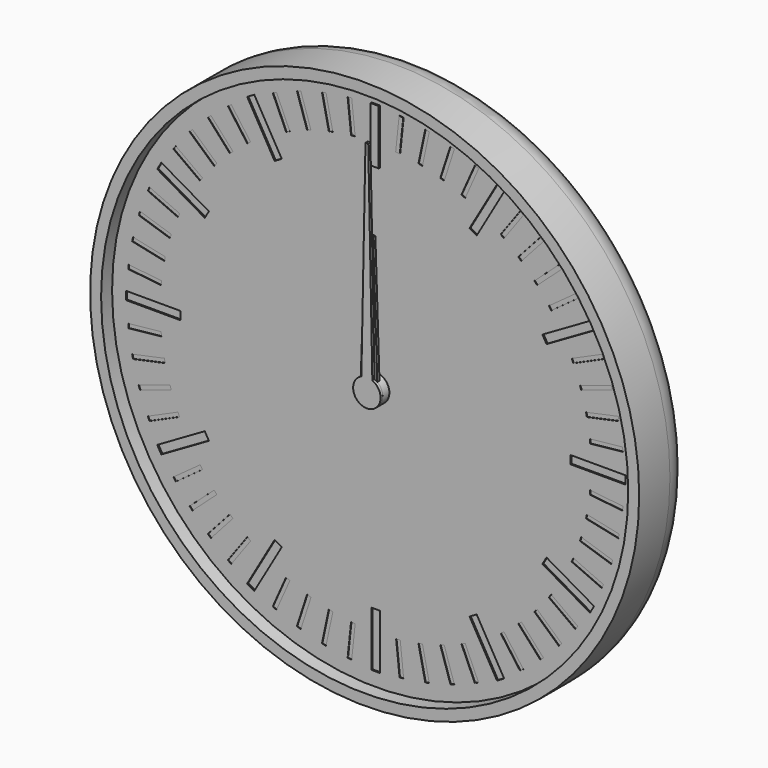
from build123d import *

# Parameters (mm, degrees)
F0_R      = 100
F1_DEPTH  = 24
F2_R      = 10
F3_T      = -4
F4_R      = 5
F4_R_2    = 3
F5_DEPTH  = 2
F6_DEPTH  = 19
F7_DEPTH  = 8
F9_DEPTH  = 4
F11_DEPTH = 4
F12_R     = 5
F12_R_2   = 3
F13_DEPTH = 2
F14_R     = 3
F15_DEPTH = 4
F17_DEPTH = 4
F18_R     = 3
F19_DEPTH = 2
F20_R     = 98
F20_R_2   = 5
F21_DEPTH = 1
F23_R     = 5
F23_R_2   = 3
F24_DEPTH = 2
F25_W     = 3
F25_H     = 20
F25_W_2   = 20
F25_H_2   = 3
F26_DEPTH = 0.5
F27_W     = 1.5
F27_H     = 12
F27_W_2   = 12
F27_H_2   = 1.5
F28_DEPTH = 0.2
F29_DEPTH = 1
F30_DEPTH = 0.4
F31_R     = 5
F31_R_2   = 3
F32_DEPTH = 5
F33_R     = 3
F34_DEPTH = 1
F36_DEPTH = 1


with BuildPart() as f1:
    # F0 (on Front) → F1 (new body)
    with BuildSketch(Plane.XZ):
        Circle(F0_R)
    extrude(amount=F1_DEPTH)

    # F2
    f2_edges = [f1.edges().sort_by_distance(p)[0] for p in [
        (-100, 0, 0),
    ]]
    fillet(f2_edges, radius=F2_R)

    # F3
    f3_openings = [f1.faces().sort_by_distance(p)[0] for p in [
        (0, -24, 0),
    ]]
    offset(amount=F3_T, openings=f3_openings)

    # F4 (on face) → F5 (join)
    with BuildSketch(Plane.XZ.offset(4)):
        Circle(F4_R)
        Circle(F4_R_2, mode=Mode.SUBTRACT)
        with Locations((40, 0)):
            Circle(F4_R)
        with Locations((40, 0)):
            Circle(F4_R_2, mode=Mode.SUBTRACT)
    extrude(amount=F5_DEPTH)


with BuildPart() as f6:
    # F6 (new): a face of the model
    f6_faces = [f1.part.faces().sort_by_distance(p)[0] for p in [
        (0, -4, 0),
    ]]
    extrude(f6_faces, amount=F6_DEPTH)

    # F8 (on face) → F9 (join)
    with BuildSketch(Plane.XZ.offset(6)):
        with BuildLine():
            ThreePointArc((9.2729637667, -1.3794085621), (9.3494561423, -0.6915886375), (9.375, 0))
            ThreePointArc((9.375, 0), (9.3494561423, 0.6915886375), (9.2729637667, 1.3794085621))
            ThreePointArc((9.2729637667, 1.3794085621), (8.9161548403, 2.8970343223), (8.3127812852, 4.3345463782))
            ThreePointArc((8.3127812852, 4.3345463782), (7.5845343223, 5.5104867402), (6.6911892658, 6.566476316))
            ThreePointArc((6.6911892658, 6.566476316), (5.5104867402, 7.5845343223), (4.1773988938, 8.3928519278))
            ThreePointArc((4.1773988938, 8.3928519278), (2.8970343223, 8.9161548403), (1.5536078905, 9.2453733036))
            ThreePointArc((1.5536078905, 9.2453733036), (0, 9.375), (-1.5536078905, 9.2453733036))
            ThreePointArc((-1.5536078905, 9.2453733036), (-2.8970343223, 8.9161548403), (-4.1773988938, 8.3928519278))
            ThreePointArc((-4.1773988938, 8.3928519278), (-5.5104867402, 7.5845343223), (-6.6911892658, 6.566476316))
            ThreePointArc((-6.6911892658, 6.566476316), (-7.5845343223, 5.5104867402), (-8.3127812852, 4.3345463782))
            ThreePointArc((-8.3127812852, 4.3345463782), (-8.9161548403, 2.8970343223), (-9.2729637667, 1.3794085621))
            ThreePointArc((-9.2729637667, 1.3794085621), (-9.375, 0), (-9.2729637667, -1.3794085621))
            ThreePointArc((-9.2729637667, -1.3794085621), (-8.9161548403, -2.8970343223), (-8.3127812852, -4.3345463782))
            ThreePointArc((-8.3127812852, -4.3345463782), (-7.5845343223, -5.5104867402), (-6.6911892658, -6.566476316))
            ThreePointArc((-6.6911892658, -6.566476316), (-5.5104867402, -7.5845343223), (-4.1773988938, -8.3928519278))
            ThreePointArc((-4.1773988938, -8.3928519278), (-2.8970343223, -8.9161548403), (-1.5536078905, -9.2453733036))
            ThreePointArc((-1.5536078905, -9.2453733036), (0, -9.375), (1.5536078905, -9.2453733036))
            ThreePointArc((1.5536078905, -9.2453733036), (2.8970343223, -8.9161548403), (4.1773988938, -8.3928519278))
            ThreePointArc((4.1773988938, -8.3928519278), (5.5104867402, -7.5845343223), (6.6911892658, -6.566476316))
            ThreePointArc((6.6911892658, -6.566476316), (7.5845343223, -5.5104867402), (8.3127812852, -4.3345463782))
            ThreePointArc((8.3127812852, -4.3345463782), (8.9161548403, -2.8970343223), (9.2729637667, -1.3794085621))
        make_face()
        with BuildLine():
            ThreePointArc((8.3127812852, 4.3345463782), (8.9161548403, 2.8970343223), (9.2729637667, 1.3794085621))
            Line((9.2729637667, 1.3794085621), (11.1823199426, 2.3946312492))
            Line((11.1823199426, 2.3946312492), (10.8182678729, 3.515068311))
            Line((10.8182678729, 3.515068311), (10.4542158031, 4.6355053728))
            Line((10.4542158031, 4.6355053728), (8.3127812852, 4.3345463782))
        make_face()
        with BuildLine():
            Line((11.1823199426, -2.3946312492), (9.2729637667, -1.3794085621))
            ThreePointArc((9.2729637667, -1.3794085621), (8.9161548403, -2.8970343223), (8.3127812852, -4.3345463782))
            Line((8.3127812852, -4.3345463782), (10.4542158031, -4.6355053728))
            Line((10.4542158031, -4.6355053728), (10.8182678729, -3.515068311))
            Line((10.8182678729, -3.515068311), (11.1823199426, -2.3946312492))
        make_face()
        with BuildLine():
            ThreePointArc((4.1773988938, 8.3928519278), (5.5104867402, 7.5845343223), (6.6911892658, 6.566476316))
            Line((6.6911892658, 6.566476316), (7.6391579371, 8.5101001246))
            Line((7.6391579371, 8.5101001246), (6.6860572448, 9.202568311))
            Line((6.6860572448, 9.202568311), (5.7329565525, 9.8950364974))
            Line((5.7329565525, 9.8950364974), (4.1773988938, 8.3928519278))
        make_face()
        with BuildLine():
            Line((7.6391579371, -8.5101001246), (6.6911892658, -6.566476316))
            ThreePointArc((6.6911892658, -6.566476316), (5.5104867402, -7.5845343223), (4.1773988938, -8.3928519278))
            Line((4.1773988938, -8.3928519278), (5.7329565525, -9.8950364974))
            Line((5.7329565525, -9.8950364974), (6.6860572448, -9.202568311))
            Line((6.6860572448, -9.202568311), (7.6391579371, -8.5101001246))
        make_face()
        with BuildLine():
            ThreePointArc((-1.5536078905, 9.2453733036), (0, 9.375), (1.5536078905, 9.2453733036))
            Line((1.5536078905, 9.2453733036), (1.1780972451, 11.375))
            Line((1.1780972451, 11.375), (0, 11.375))
            Line((0, 11.375), (-1.1780972451, 11.375))
            Line((-1.1780972451, 11.375), (-1.5536078905, 9.2453733036))
        make_face()
        with BuildLine():
            Line((1.1780972451, -11.375), (1.5536078905, -9.2453733036))
            ThreePointArc((1.5536078905, -9.2453733036), (0, -9.375), (-1.5536078905, -9.2453733036))
            Line((-1.5536078905, -9.2453733036), (-1.1780972451, -11.375))
            Line((-1.1780972451, -11.375), (0, -11.375))
            Line((0, -11.375), (1.1780972451, -11.375))
        make_face()
        with BuildLine():
            ThreePointArc((-6.6911892658, 6.566476316), (-5.5104867402, 7.5845343223), (-4.1773988938, 8.3928519278))
            Line((-4.1773988938, 8.3928519278), (-5.7329565525, 9.8950364974))
            Line((-5.7329565525, 9.8950364974), (-6.6860572448, 9.202568311))
            Line((-6.6860572448, 9.202568311), (-7.6391579371, 8.5101001246))
            Line((-7.6391579371, 8.5101001246), (-6.6911892658, 6.566476316))
        make_face()
        with BuildLine():
            Line((-5.7329565525, -9.8950364974), (-4.1773988938, -8.3928519278))
            ThreePointArc((-4.1773988938, -8.3928519278), (-5.5104867402, -7.5845343223), (-6.6911892658, -6.566476316))
            Line((-6.6911892658, -6.566476316), (-7.6391579371, -8.5101001246))
            Line((-7.6391579371, -8.5101001246), (-6.6860572448, -9.202568311))
            Line((-6.6860572448, -9.202568311), (-5.7329565525, -9.8950364974))
        make_face()
        with BuildLine():
            ThreePointArc((-9.2729637667, 1.3794085621), (-8.9161548403, 2.8970343223), (-8.3127812852, 4.3345463782))
            Line((-8.3127812852, 4.3345463782), (-10.4542158031, 4.6355053728))
            Line((-10.4542158031, 4.6355053728), (-10.8182678729, 3.515068311))
            Line((-10.8182678729, 3.515068311), (-11.1823199426, 2.3946312492))
            Line((-11.1823199426, 2.3946312492), (-9.2729637667, 1.3794085621))
        make_face()
        with BuildLine():
            Line((-10.4542158031, -4.6355053728), (-8.3127812852, -4.3345463782))
            ThreePointArc((-8.3127812852, -4.3345463782), (-8.9161548403, -2.8970343223), (-9.2729637667, -1.3794085621))
            Line((-9.2729637667, -1.3794085621), (-11.1823199426, -2.3946312492))
            Line((-11.1823199426, -2.3946312492), (-10.8182678729, -3.515068311))
            Line((-10.8182678729, -3.515068311), (-10.4542158031, -4.6355053728))
        make_face()
    extrude(amount=F9_DEPTH)

    # F35 (on face) → F36 (join)
    with BuildSketch(Plane.XZ.offset(23)):
        with BuildLine():
            ThreePointArc((-2, 4.582575695), (-2.7386127875, -4.1833001327), (5, 0))
            ThreePointArc((5, 0), (4.1833001327, 2.7386127875), (2, 4.582575695))
            ThreePointArc((2, 4.582575695), (0, 5), (-2, 4.582575695))
        make_face()
        with BuildLine():
            ThreePointArc((-2, 4.582575695), (0, 5), (2, 4.582575695))
            Line((2, 4.582575695), (0.5, 80))
            Line((0.5, 80), (0, 80))
            Line((0, 80), (-0.5, 80))
            Line((-0.5, 80), (-2, 4.582575695))
        make_face()
    extrude(amount=-F36_DEPTH)


with BuildPart() as f7:
    # F7 (new): a face of the model
    f7_faces = [f1.part.faces().sort_by_distance(p)[0] for p in [
        (40, -4, 0),
    ]]
    extrude(f7_faces, amount=F7_DEPTH)

    # F10 (on face) → F11 (join)
    with BuildSketch(Plane.XZ.offset(6)):
        with BuildLine():
            ThreePointArc((68.0831311103, -1.5340704161), (68.1145308291, -0.7673208334), (68.125, 0))
            ThreePointArc((68.125, 0), (68.1145308291, 0.7673208334), (68.0831311103, 1.5340704161))
            ThreePointArc((68.0831311103, 1.5340704161), (67.9709283072, 2.9398630294), (67.7883984907, 4.3382639757))
            ThreePointArc((67.7883984907, 4.3382639757), (67.5104012706, 5.8475163042), (67.1504961426, 7.3393585695))
            ThreePointArc((67.1504961426, 7.3393585695), (66.7484645208, 8.6911029668), (66.2791795135, 10.0209954145))
            ThreePointArc((66.2791795135, 10.0209954145), (65.6934659962, 11.4394680865), (65.0312542109, 12.8238815352))
            ThreePointArc((65.0312542109, 12.8238815352), (64.3569644814, 14.0625), (63.6214342901, 15.2657612676))
            ThreePointArc((63.6214342901, 15.2657612676), (62.7536029668, 16.5314602207), (61.8180263569, 17.747939342))
            ThreePointArc((61.8180263569, 17.747939342), (60.9009482166, 18.8192983038), (59.9313190399, 19.8433401001))
            ThreePointArc((59.9313190399, 19.8433401001), (58.8192983038, 20.9009482166), (57.6512460566, 21.8963270356))
            ThreePointArc((57.6512460566, 21.8963270356), (56.5314602207, 22.7536029668), (55.3701095067, 23.5536697513))
            ThreePointArc((55.3701095067, 23.5536697513), (54.0625, 24.3569644814), (52.7130216036, 25.0877401674))
            ThreePointArc((52.7130216036, 25.0877401674), (51.4394680865, 25.6934659962), (50.137152434, 26.2345910113))
            ThreePointArc((50.137152434, 26.2345910113), (48.6911029668, 26.7484645208), (47.2191771026, 27.1826986696))
            ThreePointArc((47.2191771026, 27.1826986696), (45.8475163042, 27.5104012706), (44.4611531566, 27.7689347566))
            ThreePointArc((44.4611531566, 27.7689347566), (42.9398630294, 27.9709283072), (41.4098199208, 28.0896428028))
            ThreePointArc((41.4098199208, 28.0896428028), (40, 28.125), (38.5901800792, 28.0896428028))
            ThreePointArc((38.5901800792, 28.0896428028), (37.0601369706, 27.9709283072), (35.5388468434, 27.7689347566))
            ThreePointArc((35.5388468434, 27.7689347566), (34.1524836958, 27.5104012706), (32.7808228974, 27.1826986696))
            ThreePointArc((32.7808228974, 27.1826986696), (31.3088970332, 26.7484645208), (29.862847566, 26.2345910113))
            ThreePointArc((29.862847566, 26.2345910113), (28.5605319135, 25.6934659962), (27.2869783964, 25.0877401674))
            ThreePointArc((27.2869783964, 25.0877401674), (25.9375, 24.3569644814), (24.6298904933, 23.5536697513))
            ThreePointArc((24.6298904933, 23.5536697513), (23.4685397793, 22.7536029668), (22.3487539434, 21.8963270356))
            ThreePointArc((22.3487539434, 21.8963270356), (21.1807016962, 20.9009482166), (20.0686809601, 19.8433401001))
            ThreePointArc((20.0686809601, 19.8433401001), (19.0990517834, 18.8192983038), (18.1819736431, 17.747939342))
            ThreePointArc((18.1819736431, 17.747939342), (17.2463970332, 16.5314602207), (16.3785657099, 15.2657612676))
            ThreePointArc((16.3785657099, 15.2657612676), (15.6430355186, 14.0625), (14.9687457891, 12.8238815352))
            ThreePointArc((14.9687457891, 12.8238815352), (14.3065340038, 11.4394680865), (13.7208204865, 10.0209954145))
            ThreePointArc((13.7208204865, 10.0209954145), (13.2515354792, 8.6911029668), (12.8495038574, 7.3393585695))
            ThreePointArc((12.8495038574, 7.3393585695), (12.4895987294, 5.8475163042), (12.2116015093, 4.3382639757))
            ThreePointArc((12.2116015093, 4.3382639757), (12.0290716928, 2.9398630294), (11.9168688897, 1.5340704161))
            ThreePointArc((11.9168688897, 1.5340704161), (11.875, 0), (11.9168688897, -1.5340704161))
            ThreePointArc((11.9168688897, -1.5340704161), (12.0290716928, -2.9398630294), (12.2116015093, -4.3382639757))
            ThreePointArc((12.2116015093, -4.3382639757), (12.4895987294, -5.8475163042), (12.8495038574, -7.3393585695))
            ThreePointArc((12.8495038574, -7.3393585695), (13.2515354792, -8.6911029668), (13.7208204865, -10.0209954145))
            ThreePointArc((13.7208204865, -10.0209954145), (14.3065340038, -11.4394680865), (14.9687457891, -12.8238815352))
            ThreePointArc((14.9687457891, -12.8238815352), (15.6430355186, -14.0625), (16.3785657099, -15.2657612676))
            ThreePointArc((16.3785657099, -15.2657612676), (17.2463970332, -16.5314602207), (18.1819736431, -17.747939342))
            ThreePointArc((18.1819736431, -17.747939342), (19.0990517834, -18.8192983038), (20.0686809601, -19.8433401001))
            ThreePointArc((20.0686809601, -19.8433401001), (21.1807016962, -20.9009482166), (22.3487539434, -21.8963270356))
            ThreePointArc((22.3487539434, -21.8963270356), (23.4685397793, -22.7536029668), (24.6298904933, -23.5536697513))
            ThreePointArc((24.6298904933, -23.5536697513), (25.9375, -24.3569644814), (27.2869783964, -25.0877401674))
            ThreePointArc((27.2869783964, -25.0877401674), (28.5605319135, -25.6934659962), (29.862847566, -26.2345910113))
            ThreePointArc((29.862847566, -26.2345910113), (31.3088970332, -26.7484645208), (32.7808228974, -27.1826986696))
            ThreePointArc((32.7808228974, -27.1826986696), (34.1524836958, -27.5104012706), (35.5388468434, -27.7689347566))
            ThreePointArc((35.5388468434, -27.7689347566), (37.0601369706, -27.9709283072), (38.5901800792, -28.0896428028))
            ThreePointArc((38.5901800792, -28.0896428028), (40, -28.125), (41.4098199208, -28.0896428028))
            ThreePointArc((41.4098199208, -28.0896428028), (42.9398630294, -27.9709283072), (44.4611531566, -27.7689347566))
            ThreePointArc((44.4611531566, -27.7689347566), (45.8475163042, -27.5104012706), (47.2191771026, -27.1826986696))
            ThreePointArc((47.2191771026, -27.1826986696), (48.6911029668, -26.7484645208), (50.137152434, -26.2345910113))
            ThreePointArc((50.137152434, -26.2345910113), (51.4394680865, -25.6934659962), (52.7130216036, -25.0877401674))
            ThreePointArc((52.7130216036, -25.0877401674), (54.0625, -24.3569644814), (55.3701095067, -23.5536697513))
            ThreePointArc((55.3701095067, -23.5536697513), (56.5314602207, -22.7536029668), (57.6512460566, -21.8963270356))
            ThreePointArc((57.6512460566, -21.8963270356), (58.8192983038, -20.9009482166), (59.9313190399, -19.8433401001))
            ThreePointArc((59.9313190399, -19.8433401001), (60.9009482166, -18.8192983038), (61.8180263569, -17.747939342))
            ThreePointArc((61.8180263569, -17.747939342), (62.7536029668, -16.5314602207), (63.6214342901, -15.2657612676))
            ThreePointArc((63.6214342901, -15.2657612676), (64.3569644814, -14.0625), (65.0312542109, -12.8238815352))
            ThreePointArc((65.0312542109, -12.8238815352), (65.6934659962, -11.4394680865), (66.2791795135, -10.0209954145))
            ThreePointArc((66.2791795135, -10.0209954145), (66.7484645208, -8.6911029668), (67.1504961426, -7.3393585695))
            ThreePointArc((67.1504961426, -7.3393585695), (67.5104012706, -5.8475163042), (67.7883984907, -4.3382639757))
            ThreePointArc((67.7883984907, -4.3382639757), (67.9709283072, -2.9398630294), (68.0831311103, -1.5340704161))
        make_face()
        with BuildLine():
            ThreePointArc((68.0831311103, 1.5340704161), (68.1145308291, 0.7673208334), (68.125, 0))
            ThreePointArc((68.125, 0), (68.1145308291, -0.7673208334), (68.0831311103, -1.5340704161))
            Line((68.0831311103, -1.5340704161), (70.1019552834, -1.1780972451))
            Line((70.1019552834, -1.1780972451), (70.1019552834, 0))
            Line((70.1019552834, 0), (70.1019552834, 1.1780972451))
            Line((70.1019552834, 1.1780972451), (68.0831311103, 1.5340704161))
        make_face()
        with BuildLine():
            ThreePointArc((67.1504961426, 7.3393585695), (67.5104012706, 5.8475163042), (67.7883984907, 4.3382639757))
            Line((67.7883984907, 4.3382639757), (69.689095528, 5.1061954262))
            Line((69.689095528, 5.1061954262), (69.4441553378, 6.2585484199))
            Line((69.4441553378, 6.2585484199), (69.1992151476, 7.4109014136))
            Line((69.1992151476, 7.4109014136), (67.1504961426, 7.3393585695))
        make_face()
        with BuildLine():
            Line((69.689095528, -5.1061954262), (67.7883984907, -4.3382639757))
            ThreePointArc((67.7883984907, -4.3382639757), (67.5104012706, -5.8475163042), (67.1504961426, -7.3393585695))
            Line((67.1504961426, -7.3393585695), (69.1992151476, -7.4109014136))
            Line((69.1992151476, -7.4109014136), (69.4441553378, -6.2585484199))
            Line((69.4441553378, -6.2585484199), (69.689095528, -5.1061954262))
        make_face()
        with BuildLine():
            ThreePointArc((65.0312542109, 12.8238815352), (65.6934659962, 11.4394680865), (66.2791795135, 10.0209954145))
            Line((66.2791795135, 10.0209954145), (67.978679834, 11.1673228551))
            Line((67.978679834, 11.1673228551), (67.4995045153, 12.243568242))
            Line((67.4995045153, 12.243568242), (67.0203291966, 13.3198136289))
            Line((67.0203291966, 13.3198136289), (65.0312542109, 12.8238815352))
        make_face()
        with BuildLine():
            Line((67.978679834, -11.1673228551), (66.2791795135, -10.0209954145))
            ThreePointArc((66.2791795135, -10.0209954145), (65.6934659962, -11.4394680865), (65.0312542109, -12.8238815352))
            Line((65.0312542109, -12.8238815352), (67.0203291966, -13.3198136289))
            Line((67.0203291966, -13.3198136289), (67.4995045153, -12.243568242))
            Line((67.4995045153, -12.243568242), (67.978679834, -11.1673228551))
        make_face()
        with BuildLine():
            ThreePointArc((61.8180263569, 17.747939342), (62.7536029668, 16.5314602207), (63.6214342901, 15.2657612676))
            Line((63.6214342901, 15.2657612676), (65.0454615746, 16.7403846884))
            Line((65.0454615746, 16.7403846884), (64.3529933881, 17.6934853807))
            Line((64.3529933881, 17.6934853807), (63.6605252017, 18.646586073))
            Line((63.6605252017, 18.646586073), (61.8180263569, 17.747939342))
        make_face()
        with BuildLine():
            Line((65.0454615746, -16.7403846884), (63.6214342901, -15.2657612676))
            ThreePointArc((63.6214342901, -15.2657612676), (62.7536029668, -16.5314602207), (61.8180263569, -17.747939342))
            Line((61.8180263569, -17.747939342), (63.6605252017, -18.646586073))
            Line((63.6605252017, -18.646586073), (64.3529933881, -17.6934853807))
            Line((64.3529933881, -17.6934853807), (65.0454615746, -16.7403846884))
        make_face()
        with BuildLine():
            ThreePointArc((57.6512460566, 21.8963270356), (58.8192983038, 20.9009482166), (59.9313190399, 19.8433401001))
            Line((59.9313190399, 19.8433401001), (61.0176364629, 21.5818113816))
            Line((61.0176364629, 21.5818113816), (60.1421395913, 22.3701123056))
            Line((60.1421395913, 22.3701123056), (59.2666427197, 23.1584132295))
            Line((59.2666427197, 23.1584132295), (57.6512460566, 21.8963270356))
        make_face()
        with BuildLine():
            Line((61.0176364629, -21.5818113816), (59.9313190399, -19.8433401001))
            ThreePointArc((59.9313190399, -19.8433401001), (58.8192983038, -20.9009482166), (57.6512460566, -21.8963270356))
            Line((57.6512460566, -21.8963270356), (59.2666427197, -23.1584132295))
            Line((59.2666427197, -23.1584132295), (60.1421395913, -22.3701123056))
            Line((60.1421395913, -22.3701123056), (61.0176364629, -21.5818113816))
        make_face()
        with BuildLine():
            ThreePointArc((52.7130216036, 25.0877401674), (54.0625, 24.3569644814), (55.3701095067, 23.5536697513))
            Line((55.3701095067, 23.5536697513), (56.0712397841, 25.4800093564))
            Line((56.0712397841, 25.4800093564), (55.0509776417, 26.069057979))
            Line((55.0509776417, 26.069057979), (54.0307154993, 26.6581066015))
            Line((54.0307154993, 26.6581066015), (52.7130216036, 25.0877401674))
        make_face()
        with BuildLine():
            Line((56.0712397841, -25.4800093564), (55.3701095067, -23.5536697513))
            ThreePointArc((55.3701095067, -23.5536697513), (54.0625, -24.3569644814), (52.7130216036, -25.0877401674))
            Line((52.7130216036, -25.0877401674), (54.0307154993, -26.6581066015))
            Line((54.0307154993, -26.6581066015), (55.0509776417, -26.069057979))
            Line((55.0509776417, -26.069057979), (56.0712397841, -25.4800093564))
        make_face()
        with BuildLine():
            ThreePointArc((47.2191771026, 27.1826986696), (48.6911029668, 26.7484645208), (50.137152434, 26.2345910113))
            Line((50.137152434, 26.2345910113), (50.4224528082, 28.2646086557))
            Line((50.4224528082, 28.2646086557), (49.3020157465, 28.6286607255))
            Line((49.3020157465, 28.6286607255), (48.1815786847, 28.9927127952))
            Line((48.1815786847, 28.9927127952), (47.2191771026, 27.1826986696))
        make_face()
        with BuildLine():
            Line((50.4224528082, -28.2646086557), (50.137152434, -26.2345910113))
            ThreePointArc((50.137152434, -26.2345910113), (48.6911029668, -26.7484645208), (47.2191771026, -27.1826986696))
            Line((47.2191771026, -27.1826986696), (48.1815786847, -28.9927127952))
            Line((48.1815786847, -28.9927127952), (49.3020157465, -28.6286607255))
            Line((49.3020157465, -28.6286607255), (50.4224528082, -28.2646086557))
        make_face()
        with BuildLine():
            ThreePointArc((41.4098199208, 28.0896428028), (42.9398630294, 27.9709283072), (44.4611531566, 27.7689347566))
            Line((44.4611531566, 27.7689347566), (44.3181546322, 29.8139089281))
            Line((44.3181546322, 29.8139089281), (43.1465111271, 29.9370536227))
            Line((43.1465111271, 29.9370536227), (41.974867622, 30.0601983173))
            Line((41.974867622, 30.0601983173), (41.4098199208, 28.0896428028))
        make_face()
        with BuildLine():
            Line((44.3181546322, -29.8139089281), (44.4611531566, -27.7689347566))
            ThreePointArc((44.4611531566, -27.7689347566), (42.9398630294, -27.9709283072), (41.4098199208, -28.0896428028))
            Line((41.4098199208, -28.0896428028), (41.974867622, -30.0601983173))
            Line((41.974867622, -30.0601983173), (43.1465111271, -29.9370536227))
            Line((43.1465111271, -29.9370536227), (44.3181546322, -29.8139089281))
        make_face()
        with BuildLine():
            ThreePointArc((35.5388468434, 27.7689347566), (37.0601369706, 27.9709283072), (38.5901800792, 28.0896428028))
            Line((38.5901800792, 28.0896428028), (38.025132378, 30.0601983173))
            Line((38.025132378, 30.0601983173), (36.8534888729, 29.9370536227))
            Line((36.8534888729, 29.9370536227), (35.6818453678, 29.8139089281))
            Line((35.6818453678, 29.8139089281), (35.5388468434, 27.7689347566))
        make_face()
        with BuildLine():
            Line((38.025132378, -30.0601983173), (38.5901800792, -28.0896428028))
            ThreePointArc((38.5901800792, -28.0896428028), (37.0601369706, -27.9709283072), (35.5388468434, -27.7689347566))
            Line((35.5388468434, -27.7689347566), (35.6818453678, -29.8139089281))
            Line((35.6818453678, -29.8139089281), (36.8534888729, -29.9370536227))
            Line((36.8534888729, -29.9370536227), (38.025132378, -30.0601983173))
        make_face()
        with BuildLine():
            ThreePointArc((29.862847566, 26.2345910113), (31.3088970332, 26.7484645208), (32.7808228974, 27.1826986696))
            Line((32.7808228974, 27.1826986696), (31.8184213153, 28.9927127952))
            Line((31.8184213153, 28.9927127952), (30.6979842535, 28.6286607255))
            Line((30.6979842535, 28.6286607255), (29.5775471918, 28.2646086557))
            Line((29.5775471918, 28.2646086557), (29.862847566, 26.2345910113))
        make_face()
        with BuildLine():
            Line((31.8184213153, -28.9927127952), (32.7808228974, -27.1826986696))
            ThreePointArc((32.7808228974, -27.1826986696), (31.3088970332, -26.7484645208), (29.862847566, -26.2345910113))
            Line((29.862847566, -26.2345910113), (29.5775471918, -28.2646086557))
            Line((29.5775471918, -28.2646086557), (30.6979842535, -28.6286607255))
            Line((30.6979842535, -28.6286607255), (31.8184213153, -28.9927127952))
        make_face()
        with BuildLine():
            ThreePointArc((24.6298904933, 23.5536697513), (25.9375, 24.3569644814), (27.2869783964, 25.0877401674))
            Line((27.2869783964, 25.0877401674), (25.9692845007, 26.6581066015))
            Line((25.9692845007, 26.6581066015), (24.9490223583, 26.069057979))
            Line((24.9490223583, 26.069057979), (23.9287602159, 25.4800093564))
            Line((23.9287602159, 25.4800093564), (24.6298904933, 23.5536697513))
        make_face()
        with BuildLine():
            Line((25.9692845007, -26.6581066015), (27.2869783964, -25.0877401674))
            ThreePointArc((27.2869783964, -25.0877401674), (25.9375, -24.3569644814), (24.6298904933, -23.5536697513))
            Line((24.6298904933, -23.5536697513), (23.9287602159, -25.4800093564))
            Line((23.9287602159, -25.4800093564), (24.9490223583, -26.069057979))
            Line((24.9490223583, -26.069057979), (25.9692845007, -26.6581066015))
        make_face()
        with BuildLine():
            ThreePointArc((20.0686809601, 19.8433401001), (21.1807016962, 20.9009482166), (22.3487539434, 21.8963270356))
            Line((22.3487539434, 21.8963270356), (20.7333572803, 23.1584132295))
            Line((20.7333572803, 23.1584132295), (19.8578604087, 22.3701123056))
            Line((19.8578604087, 22.3701123056), (18.9823635371, 21.5818113816))
            Line((18.9823635371, 21.5818113816), (20.0686809601, 19.8433401001))
        make_face()
        with BuildLine():
            Line((20.7333572803, -23.1584132295), (22.3487539434, -21.8963270356))
            ThreePointArc((22.3487539434, -21.8963270356), (21.1807016962, -20.9009482166), (20.0686809601, -19.8433401001))
            Line((20.0686809601, -19.8433401001), (18.9823635371, -21.5818113816))
            Line((18.9823635371, -21.5818113816), (19.8578604087, -22.3701123056))
            Line((19.8578604087, -22.3701123056), (20.7333572803, -23.1584132295))
        make_face()
        with BuildLine():
            ThreePointArc((16.3785657099, 15.2657612676), (17.2463970332, 16.5314602207), (18.1819736431, 17.747939342))
            Line((18.1819736431, 17.747939342), (16.3394747983, 18.646586073))
            Line((16.3394747983, 18.646586073), (15.6470066119, 17.6934853807))
            Line((15.6470066119, 17.6934853807), (14.9545384254, 16.7403846884))
            Line((14.9545384254, 16.7403846884), (16.3785657099, 15.2657612676))
        make_face()
        with BuildLine():
            Line((16.3394747983, -18.646586073), (18.1819736431, -17.747939342))
            ThreePointArc((18.1819736431, -17.747939342), (17.2463970332, -16.5314602207), (16.3785657099, -15.2657612676))
            Line((16.3785657099, -15.2657612676), (14.9545384254, -16.7403846884))
            Line((14.9545384254, -16.7403846884), (15.6470066119, -17.6934853807))
            Line((15.6470066119, -17.6934853807), (16.3394747983, -18.646586073))
        make_face()
        with BuildLine():
            ThreePointArc((13.7208204865, 10.0209954145), (14.3065340038, 11.4394680865), (14.9687457891, 12.8238815352))
            Line((14.9687457891, 12.8238815352), (12.9796708034, 13.3198136289))
            Line((12.9796708034, 13.3198136289), (12.5004954847, 12.243568242))
            Line((12.5004954847, 12.243568242), (12.021320166, 11.1673228551))
            Line((12.021320166, 11.1673228551), (13.7208204865, 10.0209954145))
        make_face()
        with BuildLine():
            Line((12.9796708034, -13.3198136289), (14.9687457891, -12.8238815352))
            ThreePointArc((14.9687457891, -12.8238815352), (14.3065340038, -11.4394680865), (13.7208204865, -10.0209954145))
            Line((13.7208204865, -10.0209954145), (12.021320166, -11.1673228551))
            Line((12.021320166, -11.1673228551), (12.5004954847, -12.243568242))
            Line((12.5004954847, -12.243568242), (12.9796708034, -13.3198136289))
        make_face()
        with BuildLine():
            ThreePointArc((12.2116015093, 4.3382639757), (12.4895987294, 5.8475163042), (12.8495038574, 7.3393585695))
            Line((12.8495038574, 7.3393585695), (10.8007848524, 7.4109014136))
            Line((10.8007848524, 7.4109014136), (10.5558446622, 6.2585484199))
            Line((10.5558446622, 6.2585484199), (10.310904472, 5.1061954262))
            Line((10.310904472, 5.1061954262), (12.2116015093, 4.3382639757))
        make_face()
        with BuildLine():
            Line((10.8007848524, -7.4109014136), (12.8495038574, -7.3393585695))
            ThreePointArc((12.8495038574, -7.3393585695), (12.4895987294, -5.8475163042), (12.2116015093, -4.3382639757))
            Line((12.2116015093, -4.3382639757), (10.310904472, -5.1061954262))
            Line((10.310904472, -5.1061954262), (10.5558446622, -6.2585484199))
            Line((10.5558446622, -6.2585484199), (10.8007848524, -7.4109014136))
        make_face()
        with BuildLine():
            ThreePointArc((11.9168688897, -1.5340704161), (11.875, 0), (11.9168688897, 1.5340704161))
            Line((11.9168688897, 1.5340704161), (9.8980447166, 1.1780972451))
            Line((9.8980447166, 1.1780972451), (9.8980447166, 0))
            Line((9.8980447166, 0), (9.8980447166, -1.1780972451))
            Line((9.8980447166, -1.1780972451), (11.9168688897, -1.5340704161))
        make_face()
    extrude(amount=F11_DEPTH)

    # F16 (on face) → F17 (join)
    with BuildSketch(Plane.XZ.offset(12)):
        with BuildLine():
            ThreePointArc((47.4288750323, -1.0304444454), (47.4821976298, -0.5164480894), (47.5, 0))
            ThreePointArc((47.5, 0), (47.4821976298, 0.5164480894), (47.4288750323, 1.0304444454))
            ThreePointArc((47.4288750323, 1.0304444454), (47.1329238722, 2.3176274578), (46.6157661985, 3.532936117))
            ThreePointArc((46.6157661985, 3.532936117), (46.0676274578, 4.4083893922), (45.4044061018, 5.2002302532))
            ThreePointArc((45.4044061018, 5.2002302532), (44.4083893922, 6.0676274578), (43.2756595386, 6.7468551628))
            ThreePointArc((43.2756595386, 6.7468551628), (42.3176274578, 7.1329238722), (41.3156377295, 7.3837048536))
            ThreePointArc((41.3156377295, 7.3837048536), (40, 7.5), (38.6843622705, 7.3837048536))
            ThreePointArc((38.6843622705, 7.3837048536), (37.6823725422, 7.1329238722), (36.7243404614, 6.7468551628))
            ThreePointArc((36.7243404614, 6.7468551628), (35.5916106078, 6.0676274578), (34.5955938982, 5.2002302532))
            ThreePointArc((34.5955938982, 5.2002302532), (33.9323725422, 4.4083893922), (33.3842338015, 3.532936117))
            ThreePointArc((33.3842338015, 3.532936117), (32.8670761278, 2.3176274578), (32.5711249677, 1.0304444454))
            ThreePointArc((32.5711249677, 1.0304444454), (32.5, 0), (32.5711249677, -1.0304444454))
            ThreePointArc((32.5711249677, -1.0304444454), (32.8670761278, -2.3176274578), (33.3842338015, -3.532936117))
            ThreePointArc((33.3842338015, -3.532936117), (33.9323725422, -4.4083893922), (34.5955938982, -5.2002302532))
            ThreePointArc((34.5955938982, -5.2002302532), (35.5916106078, -6.0676274578), (36.7243404614, -6.7468551628))
            ThreePointArc((36.7243404614, -6.7468551628), (37.6823725422, -7.1329238722), (38.6843622705, -7.3837048536))
            ThreePointArc((38.6843622705, -7.3837048536), (40, -7.5), (41.3156377295, -7.3837048536))
            ThreePointArc((41.3156377295, -7.3837048536), (42.3176274578, -7.1329238722), (43.2756595386, -6.7468551628))
            ThreePointArc((43.2756595386, -6.7468551628), (44.4083893922, -6.0676274578), (45.4044061018, -5.2002302532))
            ThreePointArc((45.4044061018, -5.2002302532), (46.0676274578, -4.4083893922), (46.6157661985, -3.532936117))
            ThreePointArc((46.6157661985, -3.532936117), (47.1329238722, -2.3176274578), (47.4288750323, -1.0304444454))
        make_face()
        with BuildLine():
            ThreePointArc((46.6157661985, 3.532936117), (47.1329238722, 2.3176274578), (47.4288750323, 1.0304444454))
            Line((47.4288750323, 1.0304444454), (49.3262785606, 2.0393117971))
            Line((49.3262785606, 2.0393117971), (48.743795249, 3.832011096))
            Line((48.743795249, 3.832011096), (46.6157661985, 3.532936117))
        make_face()
        with BuildLine():
            Line((49.3262785606, -2.0393117971), (47.4288750323, -1.0304444454))
            ThreePointArc((47.4288750323, -1.0304444454), (47.1329238722, -2.3176274578), (46.6157661985, -3.532936117))
            Line((46.6157661985, -3.532936117), (48.743795249, -3.832011096))
            Line((48.743795249, -3.832011096), (49.3262785606, -2.0393117971))
        make_face()
        with BuildLine():
            ThreePointArc((43.2756595386, 6.7468551628), (44.4083893922, 6.0676274578), (45.4044061018, 5.2002302532))
            Line((45.4044061018, 5.2002302532), (46.3464404506, 7.1316868974))
            Line((46.3464404506, 7.1316868974), (44.8214793429, 8.2396359957))
            Line((44.8214793429, 8.2396359957), (43.2756595386, 6.7468551628))
        make_face()
        with BuildLine():
            Line((46.3464404506, -7.1316868974), (45.4044061018, -5.2002302532))
            ThreePointArc((45.4044061018, -5.2002302532), (44.4083893922, -6.0676274578), (43.2756595386, -6.7468551628))
            Line((43.2756595386, -6.7468551628), (44.8214793429, -8.2396359957))
            Line((44.8214793429, -8.2396359957), (46.3464404506, -7.1316868974))
        make_face()
        with BuildLine():
            ThreePointArc((38.6843622705, 7.3837048536), (40, 7.5), (41.3156377295, 7.3837048536))
            Line((41.3156377295, 7.3837048536), (40.9424777961, 9.5))
            Line((40.9424777961, 9.5), (39.0575222039, 9.5))
            Line((39.0575222039, 9.5), (38.6843622705, 7.3837048536))
        make_face()
        with BuildLine():
            Line((40.9424777961, -9.5), (41.3156377295, -7.3837048536))
            ThreePointArc((41.3156377295, -7.3837048536), (40, -7.5), (38.6843622705, -7.3837048536))
            Line((38.6843622705, -7.3837048536), (39.0575222039, -9.5))
            Line((39.0575222039, -9.5), (40.9424777961, -9.5))
        make_face()
        with BuildLine():
            ThreePointArc((34.5955938982, 5.2002302532), (35.5916106078, 6.0676274578), (36.7243404614, 6.7468551628))
            Line((36.7243404614, 6.7468551628), (35.1785206571, 8.2396359957))
            Line((35.1785206571, 8.2396359957), (33.6535595494, 7.1316868974))
            Line((33.6535595494, 7.1316868974), (34.5955938982, 5.2002302532))
        make_face()
        with BuildLine():
            Line((35.1785206571, -8.2396359957), (36.7243404614, -6.7468551628))
            ThreePointArc((36.7243404614, -6.7468551628), (35.5916106078, -6.0676274578), (34.5955938982, -5.2002302532))
            Line((34.5955938982, -5.2002302532), (33.6535595494, -7.1316868974))
            Line((33.6535595494, -7.1316868974), (35.1785206571, -8.2396359957))
        make_face()
        with BuildLine():
            ThreePointArc((32.5711249677, 1.0304444454), (32.8670761278, 2.3176274578), (33.3842338015, 3.532936117))
            Line((33.3842338015, 3.532936117), (31.256204751, 3.832011096))
            Line((31.256204751, 3.832011096), (30.6737214394, 2.0393117971))
            Line((30.6737214394, 2.0393117971), (32.5711249677, 1.0304444454))
        make_face()
        with BuildLine():
            Line((31.256204751, -3.832011096), (33.3842338015, -3.532936117))
            ThreePointArc((33.3842338015, -3.532936117), (32.8670761278, -2.3176274578), (32.5711249677, -1.0304444454))
            Line((32.5711249677, -1.0304444454), (30.6737214394, -2.0393117971))
            Line((30.6737214394, -2.0393117971), (31.256204751, -3.832011096))
        make_face()
    extrude(amount=F17_DEPTH)

    # F18 (on face) → F19 (join)
    with BuildSketch(Plane.XZ.offset(16)):
        with Locations((40, 0)):
            Circle(F18_R)
    extrude(amount=F19_DEPTH)


with BuildPart() as f13:
    # F12 (on face) → F13 (new body)
    with BuildSketch(Plane.XZ.offset(10)):
        Circle(F12_R)
        Circle(F12_R_2, mode=Mode.SUBTRACT)
    extrude(amount=F13_DEPTH)

    # F14 (on face) → F15 (join)
    with BuildSketch(Plane.XZ.offset(12)):
        with BuildLine():
            ThreePointArc((29.9718156995, -1.3001014101), (29.9929530972, -0.6502034357), (30, 0))
            ThreePointArc((30, 0), (29.9929530972, 0.6502034357), (29.9718156995, 1.3001014101))
            ThreePointArc((29.9718156995, 1.3001014101), (29.907520012, 2.3537728718), (29.8061935814, 3.4045299509))
            ThreePointArc((29.8061935814, 3.4045299509), (29.6306502179, 4.6930339512), (29.3994322443, 5.9727199596))
            ThreePointArc((29.3994322443, 5.9727199596), (29.1710976119, 7.0033609157), (28.9066440563, 8.0253304855))
            ThreePointArc((28.9066440563, 8.0253304855), (28.5316954889, 9.2705098312), (28.1031371961, 10.4982703213))
            ThreePointArc((28.1031371961, 10.4982703213), (27.7163859753, 11.480502971), (27.2953170189, 12.448520749))
            ThreePointArc((27.2953170189, 12.448520749), (26.7301957257, 13.6197149922), (26.1148496411, 14.765318426))
            ThreePointArc((26.1148496411, 14.765318426), (25.5792049306, 15.6749569415), (25.0118886885, 16.5651871174))
            ThreePointArc((25.0118886885, 16.5651871174), (24.2705098312, 17.6335575688), (23.4835278178, 18.6687953878))
            ThreePointArc((23.4835278178, 18.6687953878), (22.812178968, 19.4834414499), (22.1125846489, 20.2739636023))
            ThreePointArc((22.1125846489, 20.2739636023), (21.2132034356, 21.2132034356), (20.2739636023, 22.1125846489))
            ThreePointArc((20.2739636023, 22.1125846489), (19.4834414499, 22.812178968), (18.6687953878, 23.4835278178))
            ThreePointArc((18.6687953878, 23.4835278178), (17.6335575688, 24.2705098312), (16.5651871174, 25.0118886885))
            ThreePointArc((16.5651871174, 25.0118886885), (15.6749569415, 25.5792049306), (14.765318426, 26.1148496411))
            ThreePointArc((14.765318426, 26.1148496411), (13.6197149922, 26.7301957257), (12.448520749, 27.2953170189))
            ThreePointArc((12.448520749, 27.2953170189), (11.480502971, 27.7163859753), (10.4982703213, 28.1031371961))
            ThreePointArc((10.4982703213, 28.1031371961), (9.2705098312, 28.5316954889), (8.0253304855, 28.9066440563))
            ThreePointArc((8.0253304855, 28.9066440563), (7.0033609157, 29.1710976119), (5.9727199596, 29.3994322443))
            ThreePointArc((5.9727199596, 29.3994322443), (4.6930339512, 29.6306502179), (3.4045299509, 29.8061935814))
            ThreePointArc((3.4045299509, 29.8061935814), (2.3537728718, 29.907520012), (1.3001014101, 29.9718156995))
            ThreePointArc((1.3001014101, 29.9718156995), (0, 30), (-1.3001014101, 29.9718156995))
            ThreePointArc((-1.3001014101, 29.9718156995), (-2.3537728718, 29.907520012), (-3.4045299509, 29.8061935814))
            ThreePointArc((-3.4045299509, 29.8061935814), (-4.6930339512, 29.6306502179), (-5.9727199596, 29.3994322443))
            ThreePointArc((-5.9727199596, 29.3994322443), (-7.0033609157, 29.1710976119), (-8.0253304855, 28.9066440563))
            ThreePointArc((-8.0253304855, 28.9066440563), (-9.2705098312, 28.5316954889), (-10.4982703213, 28.1031371961))
            ThreePointArc((-10.4982703213, 28.1031371961), (-11.480502971, 27.7163859753), (-12.448520749, 27.2953170189))
            ThreePointArc((-12.448520749, 27.2953170189), (-13.6197149922, 26.7301957257), (-14.765318426, 26.1148496411))
            ThreePointArc((-14.765318426, 26.1148496411), (-15.6749569415, 25.5792049306), (-16.5651871174, 25.0118886885))
            ThreePointArc((-16.5651871174, 25.0118886885), (-17.6335575688, 24.2705098312), (-18.6687953878, 23.4835278178))
            ThreePointArc((-18.6687953878, 23.4835278178), (-19.4834414499, 22.812178968), (-20.2739636023, 22.1125846489))
            ThreePointArc((-20.2739636023, 22.1125846489), (-21.2132034356, 21.2132034356), (-22.1125846489, 20.2739636023))
            ThreePointArc((-22.1125846489, 20.2739636023), (-22.812178968, 19.4834414499), (-23.4835278178, 18.6687953878))
            ThreePointArc((-23.4835278178, 18.6687953878), (-24.2705098312, 17.6335575688), (-25.0118886885, 16.5651871174))
            ThreePointArc((-25.0118886885, 16.5651871174), (-25.5792049306, 15.6749569415), (-26.1148496411, 14.765318426))
            ThreePointArc((-26.1148496411, 14.765318426), (-26.7301957257, 13.6197149922), (-27.2953170189, 12.448520749))
            ThreePointArc((-27.2953170189, 12.448520749), (-27.7163859753, 11.480502971), (-28.1031371961, 10.4982703213))
            ThreePointArc((-28.1031371961, 10.4982703213), (-28.5316954889, 9.2705098312), (-28.9066440563, 8.0253304855))
            ThreePointArc((-28.9066440563, 8.0253304855), (-29.1710976119, 7.0033609157), (-29.3994322443, 5.9727199596))
            ThreePointArc((-29.3994322443, 5.9727199596), (-29.6306502179, 4.6930339512), (-29.8061935814, 3.4045299509))
            ThreePointArc((-29.8061935814, 3.4045299509), (-29.907520012, 2.3537728718), (-29.9718156995, 1.3001014101))
            ThreePointArc((-29.9718156995, 1.3001014101), (-30, 0), (-29.9718156995, -1.3001014101))
            ThreePointArc((-29.9718156995, -1.3001014101), (-29.907520012, -2.3537728718), (-29.8061935814, -3.4045299509))
            ThreePointArc((-29.8061935814, -3.4045299509), (-29.6306502179, -4.6930339512), (-29.3994322443, -5.9727199596))
            ThreePointArc((-29.3994322443, -5.9727199596), (-29.1710976119, -7.0033609157), (-28.9066440563, -8.0253304855))
            ThreePointArc((-28.9066440563, -8.0253304855), (-28.5316954889, -9.2705098312), (-28.1031371961, -10.4982703213))
            ThreePointArc((-28.1031371961, -10.4982703213), (-27.7163859753, -11.480502971), (-27.2953170189, -12.448520749))
            ThreePointArc((-27.2953170189, -12.448520749), (-26.7301957257, -13.6197149922), (-26.1148496411, -14.765318426))
            ThreePointArc((-26.1148496411, -14.765318426), (-25.5792049306, -15.6749569415), (-25.0118886885, -16.5651871174))
            ThreePointArc((-25.0118886885, -16.5651871174), (-24.2705098312, -17.6335575688), (-23.4835278178, -18.6687953878))
            ThreePointArc((-23.4835278178, -18.6687953878), (-22.812178968, -19.4834414499), (-22.1125846489, -20.2739636023))
            ThreePointArc((-22.1125846489, -20.2739636023), (-21.2132034356, -21.2132034356), (-20.2739636023, -22.1125846489))
            ThreePointArc((-20.2739636023, -22.1125846489), (-19.4834414499, -22.812178968), (-18.6687953878, -23.4835278178))
            ThreePointArc((-18.6687953878, -23.4835278178), (-17.6335575688, -24.2705098312), (-16.5651871174, -25.0118886885))
            ThreePointArc((-16.5651871174, -25.0118886885), (-15.6749569415, -25.5792049306), (-14.765318426, -26.1148496411))
            ThreePointArc((-14.765318426, -26.1148496411), (-13.6197149922, -26.7301957257), (-12.448520749, -27.2953170189))
            ThreePointArc((-12.448520749, -27.2953170189), (-11.480502971, -27.7163859753), (-10.4982703213, -28.1031371961))
            ThreePointArc((-10.4982703213, -28.1031371961), (-9.2705098312, -28.5316954889), (-8.0253304855, -28.9066440563))
            ThreePointArc((-8.0253304855, -28.9066440563), (-7.0033609157, -29.1710976119), (-5.9727199596, -29.3994322443))
            ThreePointArc((-5.9727199596, -29.3994322443), (-4.6930339512, -29.6306502179), (-3.4045299509, -29.8061935814))
            ThreePointArc((-3.4045299509, -29.8061935814), (-2.3537728718, -29.907520012), (-1.3001014101, -29.9718156995))
            ThreePointArc((-1.3001014101, -29.9718156995), (0, -30), (1.3001014101, -29.9718156995))
            ThreePointArc((1.3001014101, -29.9718156995), (2.3537728718, -29.907520012), (3.4045299509, -29.8061935814))
            ThreePointArc((3.4045299509, -29.8061935814), (4.6930339512, -29.6306502179), (5.9727199596, -29.3994322443))
            ThreePointArc((5.9727199596, -29.3994322443), (7.0033609157, -29.1710976119), (8.0253304855, -28.9066440563))
            ThreePointArc((8.0253304855, -28.9066440563), (9.2705098312, -28.5316954889), (10.4982703213, -28.1031371961))
            ThreePointArc((10.4982703213, -28.1031371961), (11.480502971, -27.7163859753), (12.448520749, -27.2953170189))
            ThreePointArc((12.448520749, -27.2953170189), (13.6197149922, -26.7301957257), (14.765318426, -26.1148496411))
            ThreePointArc((14.765318426, -26.1148496411), (15.6749569415, -25.5792049306), (16.5651871174, -25.0118886885))
            ThreePointArc((16.5651871174, -25.0118886885), (17.6335575688, -24.2705098312), (18.6687953878, -23.4835278178))
            ThreePointArc((18.6687953878, -23.4835278178), (19.4834414499, -22.812178968), (20.2739636023, -22.1125846489))
            ThreePointArc((20.2739636023, -22.1125846489), (21.2132034356, -21.2132034356), (22.1125846489, -20.2739636023))
            ThreePointArc((22.1125846489, -20.2739636023), (22.812178968, -19.4834414499), (23.4835278178, -18.6687953878))
            ThreePointArc((23.4835278178, -18.6687953878), (24.2705098312, -17.6335575688), (25.0118886885, -16.5651871174))
            ThreePointArc((25.0118886885, -16.5651871174), (25.5792049306, -15.6749569415), (26.1148496411, -14.765318426))
            ThreePointArc((26.1148496411, -14.765318426), (26.7301957257, -13.6197149922), (27.2953170189, -12.448520749))
            ThreePointArc((27.2953170189, -12.448520749), (27.7163859753, -11.480502971), (28.1031371961, -10.4982703213))
            ThreePointArc((28.1031371961, -10.4982703213), (28.5316954889, -9.2705098312), (28.9066440563, -8.0253304855))
            ThreePointArc((28.9066440563, -8.0253304855), (29.1710976119, -7.0033609157), (29.3994322443, -5.9727199596))
            ThreePointArc((29.3994322443, -5.9727199596), (29.6306502179, -4.6930339512), (29.8061935814, -3.4045299509))
            ThreePointArc((29.8061935814, -3.4045299509), (29.907520012, -2.3537728718), (29.9718156995, -1.3001014101))
        make_face()
        Circle(F14_R, mode=Mode.SUBTRACT)
        with BuildLine():
            ThreePointArc((29.9718156995, 1.3001014101), (29.9929530972, 0.6502034357), (30, 0))
            ThreePointArc((30, 0), (29.9929530972, -0.6502034357), (29.9718156995, -1.3001014101))
            Line((29.9718156995, -1.3001014101), (32, -0.9424777961))
            Line((32, -0.9424777961), (32, 0))
            Line((32, 0), (32, 0.9424777961))
            Line((32, 0.9424777961), (29.9718156995, 1.3001014101))
        make_face()
        with BuildLine():
            ThreePointArc((29.3994322443, 5.9727199596), (29.6306502179, 4.6930339512), (29.8061935814, 3.4045299509))
            Line((29.8061935814, 3.4045299509), (31.7534629089, 4.0750285508))
            Line((31.7534629089, 4.0750285508), (31.606026899, 5.0059028813))
            Line((31.606026899, 5.0059028813), (31.4585908892, 5.9367772117))
            Line((31.4585908892, 5.9367772117), (29.3994322443, 5.9727199596))
        make_face()
        with BuildLine():
            Line((31.7534629089, -4.0750285508), (29.8061935814, -3.4045299509))
            ThreePointArc((29.8061935814, -3.4045299509), (29.6306502179, -4.6930339512), (29.3994322443, -5.9727199596))
            Line((29.3994322443, -5.9727199596), (31.4585908892, -5.9367772117))
            Line((31.4585908892, -5.9367772117), (31.606026899, -5.0059028813))
            Line((31.606026899, -5.0059028813), (31.7534629089, -4.0750285508))
        make_face()
        with BuildLine():
            ThreePointArc((28.1031371961, 10.4982703213), (28.5316954889, 9.2705098312), (28.9066440563, 8.0253304855))
            Line((28.9066440563, 8.0253304855), (30.7250501773, 8.9921941706))
            Line((30.7250501773, 8.9921941706), (30.4338085214, 9.88854382))
            Line((30.4338085214, 9.88854382), (30.1425668656, 10.7848934694))
            Line((30.1425668656, 10.7848934694), (28.1031371961, 10.4982703213))
        make_face()
        with BuildLine():
            Line((30.7250501773, -8.9921941706), (28.9066440563, -8.0253304855))
            ThreePointArc((28.9066440563, -8.0253304855), (28.5316954889, -9.2705098312), (28.1031371961, -10.4982703213))
            Line((28.1031371961, -10.4982703213), (30.1425668656, -10.7848934694))
            Line((30.1425668656, -10.7848934694), (30.4338085214, -9.88854382))
            Line((30.4338085214, -9.88854382), (30.7250501773, -8.9921941706))
        make_face()
        with BuildLine():
            ThreePointArc((26.1148496411, 14.765318426), (26.7301957257, 13.6197149922), (27.2953170189, 12.448520749))
            Line((27.2953170189, 12.448520749), (28.9400847397, 13.6879421265))
            Line((28.9400847397, 13.6879421265), (28.512208774, 14.5276959917))
            Line((28.512208774, 14.5276959917), (28.0843328084, 15.3674498569))
            Line((28.0843328084, 15.3674498569), (26.1148496411, 14.765318426))
        make_face()
        with BuildLine():
            Line((28.9400847397, -13.6879421265), (27.2953170189, -12.448520749))
            ThreePointArc((27.2953170189, -12.448520749), (26.7301957257, -13.6197149922), (26.1148496411, -14.765318426))
            Line((26.1148496411, -14.765318426), (28.0843328084, -15.3674498569))
            Line((28.0843328084, -15.3674498569), (28.512208774, -14.5276959917))
            Line((28.512208774, -14.5276959917), (28.9400847397, -13.6879421265))
        make_face()
        with BuildLine():
            ThreePointArc((23.4835278178, 18.6687953878), (24.2705098312, 17.6335575688), (25.0118886885, 16.5651871174))
            Line((25.0118886885, 16.5651871174), (26.4425183691, 18.0466475195))
            Line((26.4425183691, 18.0466475195), (25.88854382, 18.8091280734))
            Line((25.88854382, 18.8091280734), (25.3345692709, 19.5716086272))
            Line((25.3345692709, 19.5716086272), (23.4835278178, 18.6687953878))
        make_face()
        with BuildLine():
            Line((26.4425183691, -18.0466475195), (25.0118886885, -16.5651871174))
            ThreePointArc((25.0118886885, -16.5651871174), (24.2705098312, -17.6335575688), (23.4835278178, -18.6687953878))
            Line((23.4835278178, -18.6687953878), (25.3345692709, -19.5716086272))
            Line((25.3345692709, -19.5716086272), (25.88854382, -18.8091280734))
            Line((25.88854382, -18.8091280734), (26.4425183691, -18.0466475195))
        make_face()
        with BuildLine():
            ThreePointArc((20.2739636023, 22.1125846489), (21.2132034356, 21.2132034356), (22.1125846489, 20.2739636023))
            Line((22.1125846489, 20.2739636023), (23.2938494387, 21.9609845572))
            Line((23.2938494387, 21.9609845572), (22.627416998, 22.627416998))
            Line((22.627416998, 22.627416998), (21.9609845572, 23.2938494387))
            Line((21.9609845572, 23.2938494387), (20.2739636023, 22.1125846489))
        make_face()
        with BuildLine():
            Line((23.2938494387, -21.9609845572), (22.1125846489, -20.2739636023))
            ThreePointArc((22.1125846489, -20.2739636023), (21.2132034356, -21.2132034356), (20.2739636023, -22.1125846489))
            Line((20.2739636023, -22.1125846489), (21.9609845572, -23.2938494387))
            Line((21.9609845572, -23.2938494387), (22.627416998, -22.627416998))
            Line((22.627416998, -22.627416998), (23.2938494387, -21.9609845572))
        make_face()
        with BuildLine():
            ThreePointArc((16.5651871174, 25.0118886885), (17.6335575688, 24.2705098312), (18.6687953878, 23.4835278178))
            Line((18.6687953878, 23.4835278178), (19.5716086272, 25.3345692709))
            Line((19.5716086272, 25.3345692709), (18.8091280734, 25.88854382))
            Line((18.8091280734, 25.88854382), (18.0466475195, 26.4425183691))
            Line((18.0466475195, 26.4425183691), (16.5651871174, 25.0118886885))
        make_face()
        with BuildLine():
            Line((19.5716086272, -25.3345692709), (18.6687953878, -23.4835278178))
            ThreePointArc((18.6687953878, -23.4835278178), (17.6335575688, -24.2705098312), (16.5651871174, -25.0118886885))
            Line((16.5651871174, -25.0118886885), (18.0466475195, -26.4425183691))
            Line((18.0466475195, -26.4425183691), (18.8091280734, -25.88854382))
            Line((18.8091280734, -25.88854382), (19.5716086272, -25.3345692709))
        make_face()
        with BuildLine():
            ThreePointArc((12.448520749, 27.2953170189), (13.6197149922, 26.7301957257), (14.765318426, 26.1148496411))
            Line((14.765318426, 26.1148496411), (15.3674498569, 28.0843328084))
            Line((15.3674498569, 28.0843328084), (14.5276959917, 28.512208774))
            Line((14.5276959917, 28.512208774), (13.6879421265, 28.9400847397))
            Line((13.6879421265, 28.9400847397), (12.448520749, 27.2953170189))
        make_face()
        with BuildLine():
            Line((15.3674498569, -28.0843328084), (14.765318426, -26.1148496411))
            ThreePointArc((14.765318426, -26.1148496411), (13.6197149922, -26.7301957257), (12.448520749, -27.2953170189))
            Line((12.448520749, -27.2953170189), (13.6879421265, -28.9400847397))
            Line((13.6879421265, -28.9400847397), (14.5276959917, -28.512208774))
            Line((14.5276959917, -28.512208774), (15.3674498569, -28.0843328084))
        make_face()
        with BuildLine():
            ThreePointArc((8.0253304855, 28.9066440563), (9.2705098312, 28.5316954889), (10.4982703213, 28.1031371961))
            Line((10.4982703213, 28.1031371961), (10.7848934694, 30.1425668656))
            Line((10.7848934694, 30.1425668656), (9.88854382, 30.4338085214))
            Line((9.88854382, 30.4338085214), (8.9921941706, 30.7250501773))
            Line((8.9921941706, 30.7250501773), (8.0253304855, 28.9066440563))
        make_face()
        with BuildLine():
            Line((10.7848934694, -30.1425668656), (10.4982703213, -28.1031371961))
            ThreePointArc((10.4982703213, -28.1031371961), (9.2705098312, -28.5316954889), (8.0253304855, -28.9066440563))
            Line((8.0253304855, -28.9066440563), (8.9921941706, -30.7250501773))
            Line((8.9921941706, -30.7250501773), (9.88854382, -30.4338085214))
            Line((9.88854382, -30.4338085214), (10.7848934694, -30.1425668656))
        make_face()
        with BuildLine():
            ThreePointArc((3.4045299509, 29.8061935814), (4.6930339512, 29.6306502179), (5.9727199596, 29.3994322443))
            Line((5.9727199596, 29.3994322443), (5.9367772117, 31.4585908892))
            Line((5.9367772117, 31.4585908892), (5.0059028813, 31.606026899))
            Line((5.0059028813, 31.606026899), (4.0750285508, 31.7534629089))
            Line((4.0750285508, 31.7534629089), (3.4045299509, 29.8061935814))
        make_face()
        with BuildLine():
            Line((5.9367772117, -31.4585908892), (5.9727199596, -29.3994322443))
            ThreePointArc((5.9727199596, -29.3994322443), (4.6930339512, -29.6306502179), (3.4045299509, -29.8061935814))
            Line((3.4045299509, -29.8061935814), (4.0750285508, -31.7534629089))
            Line((4.0750285508, -31.7534629089), (5.0059028813, -31.606026899))
            Line((5.0059028813, -31.606026899), (5.9367772117, -31.4585908892))
        make_face()
        with BuildLine():
            ThreePointArc((-1.3001014101, 29.9718156995), (0, 30), (1.3001014101, 29.9718156995))
            Line((1.3001014101, 29.9718156995), (0.9424777961, 32))
            Line((0.9424777961, 32), (0, 32))
            Line((0, 32), (-0.9424777961, 32))
            Line((-0.9424777961, 32), (-1.3001014101, 29.9718156995))
        make_face()
        with BuildLine():
            Line((0.9424777961, -32), (1.3001014101, -29.9718156995))
            ThreePointArc((1.3001014101, -29.9718156995), (0, -30), (-1.3001014101, -29.9718156995))
            Line((-1.3001014101, -29.9718156995), (-0.9424777961, -32))
            Line((-0.9424777961, -32), (0, -32))
            Line((0, -32), (0.9424777961, -32))
        make_face()
        with BuildLine():
            ThreePointArc((-5.9727199596, 29.3994322443), (-4.6930339512, 29.6306502179), (-3.4045299509, 29.8061935814))
            Line((-3.4045299509, 29.8061935814), (-4.0750285508, 31.7534629089))
            Line((-4.0750285508, 31.7534629089), (-5.0059028813, 31.606026899))
            Line((-5.0059028813, 31.606026899), (-5.9367772117, 31.4585908892))
            Line((-5.9367772117, 31.4585908892), (-5.9727199596, 29.3994322443))
        make_face()
        with BuildLine():
            Line((-4.0750285508, -31.7534629089), (-3.4045299509, -29.8061935814))
            ThreePointArc((-3.4045299509, -29.8061935814), (-4.6930339512, -29.6306502179), (-5.9727199596, -29.3994322443))
            Line((-5.9727199596, -29.3994322443), (-5.9367772117, -31.4585908892))
            Line((-5.9367772117, -31.4585908892), (-5.0059028813, -31.606026899))
            Line((-5.0059028813, -31.606026899), (-4.0750285508, -31.7534629089))
        make_face()
        with BuildLine():
            ThreePointArc((-10.4982703213, 28.1031371961), (-9.2705098312, 28.5316954889), (-8.0253304855, 28.9066440563))
            Line((-8.0253304855, 28.9066440563), (-8.9921941706, 30.7250501773))
            Line((-8.9921941706, 30.7250501773), (-9.88854382, 30.4338085214))
            Line((-9.88854382, 30.4338085214), (-10.7848934694, 30.1425668656))
            Line((-10.7848934694, 30.1425668656), (-10.4982703213, 28.1031371961))
        make_face()
        with BuildLine():
            Line((-8.9921941706, -30.7250501773), (-8.0253304855, -28.9066440563))
            ThreePointArc((-8.0253304855, -28.9066440563), (-9.2705098312, -28.5316954889), (-10.4982703213, -28.1031371961))
            Line((-10.4982703213, -28.1031371961), (-10.7848934694, -30.1425668656))
            Line((-10.7848934694, -30.1425668656), (-9.88854382, -30.4338085214))
            Line((-9.88854382, -30.4338085214), (-8.9921941706, -30.7250501773))
        make_face()
        with BuildLine():
            ThreePointArc((-14.765318426, 26.1148496411), (-13.6197149922, 26.7301957257), (-12.448520749, 27.2953170189))
            Line((-12.448520749, 27.2953170189), (-13.6879421265, 28.9400847397))
            Line((-13.6879421265, 28.9400847397), (-14.5276959917, 28.512208774))
            Line((-14.5276959917, 28.512208774), (-15.3674498569, 28.0843328084))
            Line((-15.3674498569, 28.0843328084), (-14.765318426, 26.1148496411))
        make_face()
        with BuildLine():
            Line((-13.6879421265, -28.9400847397), (-12.448520749, -27.2953170189))
            ThreePointArc((-12.448520749, -27.2953170189), (-13.6197149922, -26.7301957257), (-14.765318426, -26.1148496411))
            Line((-14.765318426, -26.1148496411), (-15.3674498569, -28.0843328084))
            Line((-15.3674498569, -28.0843328084), (-14.5276959917, -28.512208774))
            Line((-14.5276959917, -28.512208774), (-13.6879421265, -28.9400847397))
        make_face()
        with BuildLine():
            ThreePointArc((-18.6687953878, 23.4835278178), (-17.6335575688, 24.2705098312), (-16.5651871174, 25.0118886885))
            Line((-16.5651871174, 25.0118886885), (-18.0466475195, 26.4425183691))
            Line((-18.0466475195, 26.4425183691), (-18.8091280734, 25.88854382))
            Line((-18.8091280734, 25.88854382), (-19.5716086272, 25.3345692709))
            Line((-19.5716086272, 25.3345692709), (-18.6687953878, 23.4835278178))
        make_face()
        with BuildLine():
            Line((-18.0466475195, -26.4425183691), (-16.5651871174, -25.0118886885))
            ThreePointArc((-16.5651871174, -25.0118886885), (-17.6335575688, -24.2705098312), (-18.6687953878, -23.4835278178))
            Line((-18.6687953878, -23.4835278178), (-19.5716086272, -25.3345692709))
            Line((-19.5716086272, -25.3345692709), (-18.8091280734, -25.88854382))
            Line((-18.8091280734, -25.88854382), (-18.0466475195, -26.4425183691))
        make_face()
        with BuildLine():
            ThreePointArc((-22.1125846489, 20.2739636023), (-21.2132034356, 21.2132034356), (-20.2739636023, 22.1125846489))
            Line((-20.2739636023, 22.1125846489), (-21.9609845572, 23.2938494387))
            Line((-21.9609845572, 23.2938494387), (-22.627416998, 22.627416998))
            Line((-22.627416998, 22.627416998), (-23.2938494387, 21.9609845572))
            Line((-23.2938494387, 21.9609845572), (-22.1125846489, 20.2739636023))
        make_face()
        with BuildLine():
            Line((-21.9609845572, -23.2938494387), (-20.2739636023, -22.1125846489))
            ThreePointArc((-20.2739636023, -22.1125846489), (-21.2132034356, -21.2132034356), (-22.1125846489, -20.2739636023))
            Line((-22.1125846489, -20.2739636023), (-23.2938494387, -21.9609845572))
            Line((-23.2938494387, -21.9609845572), (-22.627416998, -22.627416998))
            Line((-22.627416998, -22.627416998), (-21.9609845572, -23.2938494387))
        make_face()
        with BuildLine():
            ThreePointArc((-25.0118886885, 16.5651871174), (-24.2705098312, 17.6335575688), (-23.4835278178, 18.6687953878))
            Line((-23.4835278178, 18.6687953878), (-25.3345692709, 19.5716086272))
            Line((-25.3345692709, 19.5716086272), (-25.88854382, 18.8091280734))
            Line((-25.88854382, 18.8091280734), (-26.4425183691, 18.0466475195))
            Line((-26.4425183691, 18.0466475195), (-25.0118886885, 16.5651871174))
        make_face()
        with BuildLine():
            Line((-25.3345692709, -19.5716086272), (-23.4835278178, -18.6687953878))
            ThreePointArc((-23.4835278178, -18.6687953878), (-24.2705098312, -17.6335575688), (-25.0118886885, -16.5651871174))
            Line((-25.0118886885, -16.5651871174), (-26.4425183691, -18.0466475195))
            Line((-26.4425183691, -18.0466475195), (-25.88854382, -18.8091280734))
            Line((-25.88854382, -18.8091280734), (-25.3345692709, -19.5716086272))
        make_face()
        with BuildLine():
            ThreePointArc((-27.2953170189, 12.448520749), (-26.7301957257, 13.6197149922), (-26.1148496411, 14.765318426))
            Line((-26.1148496411, 14.765318426), (-28.0843328084, 15.3674498569))
            Line((-28.0843328084, 15.3674498569), (-28.512208774, 14.5276959917))
            Line((-28.512208774, 14.5276959917), (-28.9400847397, 13.6879421265))
            Line((-28.9400847397, 13.6879421265), (-27.2953170189, 12.448520749))
        make_face()
        with BuildLine():
            Line((-28.0843328084, -15.3674498569), (-26.1148496411, -14.765318426))
            ThreePointArc((-26.1148496411, -14.765318426), (-26.7301957257, -13.6197149922), (-27.2953170189, -12.448520749))
            Line((-27.2953170189, -12.448520749), (-28.9400847397, -13.6879421265))
            Line((-28.9400847397, -13.6879421265), (-28.512208774, -14.5276959917))
            Line((-28.512208774, -14.5276959917), (-28.0843328084, -15.3674498569))
        make_face()
        with BuildLine():
            ThreePointArc((-28.9066440563, 8.0253304855), (-28.5316954889, 9.2705098312), (-28.1031371961, 10.4982703213))
            Line((-28.1031371961, 10.4982703213), (-30.1425668656, 10.7848934694))
            Line((-30.1425668656, 10.7848934694), (-30.4338085214, 9.88854382))
            Line((-30.4338085214, 9.88854382), (-30.7250501773, 8.9921941706))
            Line((-30.7250501773, 8.9921941706), (-28.9066440563, 8.0253304855))
        make_face()
        with BuildLine():
            Line((-30.1425668656, -10.7848934694), (-28.1031371961, -10.4982703213))
            ThreePointArc((-28.1031371961, -10.4982703213), (-28.5316954889, -9.2705098312), (-28.9066440563, -8.0253304855))
            Line((-28.9066440563, -8.0253304855), (-30.7250501773, -8.9921941706))
            Line((-30.7250501773, -8.9921941706), (-30.4338085214, -9.88854382))
            Line((-30.4338085214, -9.88854382), (-30.1425668656, -10.7848934694))
        make_face()
        with BuildLine():
            ThreePointArc((-29.8061935814, 3.4045299509), (-29.6306502179, 4.6930339512), (-29.3994322443, 5.9727199596))
            Line((-29.3994322443, 5.9727199596), (-31.4585908892, 5.9367772117))
            Line((-31.4585908892, 5.9367772117), (-31.606026899, 5.0059028813))
            Line((-31.606026899, 5.0059028813), (-31.7534629089, 4.0750285508))
            Line((-31.7534629089, 4.0750285508), (-29.8061935814, 3.4045299509))
        make_face()
        with BuildLine():
            Line((-31.4585908892, -5.9367772117), (-29.3994322443, -5.9727199596))
            ThreePointArc((-29.3994322443, -5.9727199596), (-29.6306502179, -4.6930339512), (-29.8061935814, -3.4045299509))
            Line((-29.8061935814, -3.4045299509), (-31.7534629089, -4.0750285508))
            Line((-31.7534629089, -4.0750285508), (-31.606026899, -5.0059028813))
            Line((-31.606026899, -5.0059028813), (-31.4585908892, -5.9367772117))
        make_face()
        with BuildLine():
            ThreePointArc((-29.9718156995, -1.3001014101), (-30, 0), (-29.9718156995, 1.3001014101))
            Line((-29.9718156995, 1.3001014101), (-32, 0.9424777961))
            Line((-32, 0.9424777961), (-32, 0))
            Line((-32, 0), (-32, -0.9424777961))
            Line((-32, -0.9424777961), (-29.9718156995, -1.3001014101))
        make_face()
    extrude(amount=F15_DEPTH)

    # F31 (on face) → F32 (join)
    with BuildSketch(Plane.XZ.offset(16)):
        Circle(F31_R)
        Circle(F31_R_2, mode=Mode.SUBTRACT)
    extrude(amount=F32_DEPTH)

    # F33 (on face) → F34 (join)
    with BuildSketch(Plane.XZ.offset(21)):
        with BuildLine():
            Line((1.5, 50), (0, 50))
            Line((0, 50), (-1.5, 50))
            Line((-1.5, 50), (-3, 4))
            ThreePointArc((-3, 4), (0, 5), (3, 4))
            Line((3, 4), (1.5, 50))
        make_face()
        with BuildLine():
            ThreePointArc((5, 0), (4.472135955, 2.2360679775), (3, 4))
            ThreePointArc((3, 4), (0, 5), (-3, 4))
            ThreePointArc((-3, 4), (-2.2360679775, -4.472135955), (5, 0))
        make_face()
        Circle(F33_R, mode=Mode.SUBTRACT)
    extrude(amount=F34_DEPTH)


with BuildPart() as f21:
    # F20 (on face) → F21 (new body)
    with BuildSketch(Plane.XZ.offset(18)):
        Circle(F20_R)
        Circle(F20_R_2, mode=Mode.SUBTRACT)
    extrude(amount=F21_DEPTH)


with BuildPart() as f1_1:
    add(f1.part)

    # F22: cut F21
    add(f21.part, mode=Mode.SUBTRACT)


with BuildPart() as f21_1:
    add(f21.part)

    # F23 (on face) → F24 (join, through all)
    with BuildSketch(Plane(origin=(0, -18, 0), x_dir=(-1, 0, 0), z_dir=(0, 1, 0))):
        with Locations((-40, 0)):
            Circle(F23_R)
        with Locations((-40, 0)):
            Circle(F23_R_2, mode=Mode.SUBTRACT)
    extrude(amount=F24_DEPTH)

    # F25 (on face) → F26 (cut)
    with BuildSketch(Plane.XZ.offset(19)):
        with Locations((0, 81)):
            Rectangle(F25_W, F25_H)
        Polygon((-34.2009618943, 62.2378036687), (-44.2009618943, 79.5583117444), (-46.7990381057, 78.0583117444), (-36.7990381057, 60.7378036687), align=None)
        Polygon((-60.7378036687, 36.7990381057), (-78.0583117444, 46.7990381057), (-79.5583117444, 44.2009618943), (-62.2378036687, 34.2009618943), align=None)
        with Locations((-81, 0)):
            Rectangle(F25_W_2, F25_H_2)
        Polygon((-62.2378036687, -34.2009618943), (-79.5583117444, -44.2009618943), (-78.0583117444, -46.7990381057), (-60.7378036687, -36.7990381057), align=None)
        Polygon((-36.7990381057, -60.7378036687), (-46.7990381057, -78.0583117444), (-44.2009618943, -79.5583117444), (-34.2009618943, -62.2378036687), align=None)
        with Locations((0, -81)):
            Rectangle(F25_W, F25_H)
        Polygon((34.2009618943, -62.2378036687), (44.2009618943, -79.5583117444), (46.7990381057, -78.0583117444), (36.7990381057, -60.7378036687), align=None)
        Polygon((60.7378036687, -36.7990381057), (78.0583117444, -46.7990381057), (79.5583117444, -44.2009618943), (62.2378036687, -34.2009618943), align=None)
        with Locations((81, 0)):
            Rectangle(F25_W_2, F25_H_2)
        Polygon((62.2378036687, 34.2009618943), (79.5583117444, 44.2009618943), (78.0583117444, 46.7990381057), (60.7378036687, 36.7990381057), align=None)
        Polygon((36.7990381057, 60.7378036687), (46.7990381057, 78.0583117444), (44.2009618943, 79.5583117444), (34.2009618943, 62.2378036687), align=None)
    extrude(amount=-F26_DEPTH, mode=Mode.SUBTRACT)

    # F27 (on face) → F28 (cut)
    with BuildSketch(Plane.XZ.offset(19)):
        with Locations((0, 84.5)):
            Rectangle(F27_W, F27_H)
        Polygon((-7.459592945, 78.1483651339), (-8.7139345042, 90.0826278783), (-10.2057173472, 89.9258351834), (-8.951375788, 77.991572439), align=None)
        Polygon((-15.5874570286, 76.9405204257), (-18.0823973185, 88.6782916345), (-19.5496187196, 88.3664240983), (-17.0546784297, 76.6286528895), align=None)
        Polygon((-23.5445416712, 74.889699275), (-27.2527456037, 86.3023774705), (-28.6793303782, 85.8388519789), (-24.9711264457, 74.4261737834), align=None)
        Polygon((-31.2436673882, 72.0183709073), (-36.1245071051, 82.980916399), (-37.4948252916, 82.3708114343), (-32.6139855747, 71.4082659426), align=None)
        Polygon((-38.6004809472, 68.3579941971), (-44.6004809472, 78.7502990425), (-45.8995190528, 78.0002990425), (-39.8995190528, 67.6079941971), align=None)
        Polygon((-45.5343795592, 63.9486729977), (-52.5878025867, 73.6568769302), (-53.8013280783, 72.7751990517), (-46.7479050507, 63.0669951192), align=None)
        Polygon((-51.9693939801, 58.8387167547), (-59.9989612564, 67.7564546605), (-61.1136784946, 66.7527587509), (-53.0841112183, 57.8350208452), align=None)
        Polygon((-57.8350208452, 53.0841112183), (-66.7527587509, 61.1136784946), (-67.7564546605, 59.9989612564), (-58.8387167547, 51.9693939801), align=None)
        Polygon((-63.0669951192, 46.7479050507), (-72.7751990517, 53.8013280783), (-73.6568769302, 52.5878025867), (-63.9486729977, 45.5343795592), align=None)
        Polygon((-67.6079941971, 39.8995190528), (-78.0002990425, 45.8995190528), (-78.7502990425, 44.6004809472), (-68.3579941971, 38.6004809472), align=None)
        Polygon((-71.4082659426, 32.6139855747), (-82.3708114343, 37.4948252916), (-82.980916399, 36.1245071051), (-72.0183709073, 31.2436673882), align=None)
        Polygon((-74.4261737834, 24.9711264457), (-85.8388519789, 28.6793303782), (-86.3023774705, 27.2527456037), (-74.889699275, 23.5445416712), align=None)
        Polygon((-76.6286528895, 17.0546784297), (-88.3664240983, 19.5496187196), (-88.6782916345, 18.0823973185), (-76.9405204257, 15.5874570286), align=None)
        Polygon((-77.991572439, 8.951375788), (-89.9258351834, 10.2057173472), (-90.0826278783, 8.7139345042), (-78.1483651339, 7.459592945), align=None)
        with Locations((-84.5, 0)):
            Rectangle(F27_W_2, F27_H_2)
        Polygon((-78.1483651339, -7.459592945), (-90.0826278783, -8.7139345042), (-89.9258351834, -10.2057173472), (-77.991572439, -8.951375788), align=None)
        Polygon((-76.9405204257, -15.5874570286), (-88.6782916345, -18.0823973185), (-88.3664240983, -19.5496187196), (-76.6286528895, -17.0546784297), align=None)
        Polygon((-74.889699275, -23.5445416712), (-86.3023774705, -27.2527456037), (-85.8388519789, -28.6793303782), (-74.4261737834, -24.9711264457), align=None)
        Polygon((-72.0183709073, -31.2436673882), (-82.980916399, -36.1245071051), (-82.3708114343, -37.4948252916), (-71.4082659426, -32.6139855747), align=None)
        Polygon((-68.3579941971, -38.6004809472), (-78.7502990425, -44.6004809472), (-78.0002990425, -45.8995190528), (-67.6079941971, -39.8995190528), align=None)
        Polygon((-63.9486729977, -45.5343795592), (-73.6568769302, -52.5878025867), (-72.7751990517, -53.8013280783), (-63.0669951192, -46.7479050507), align=None)
        Polygon((-58.8387167547, -51.9693939801), (-67.7564546605, -59.9989612564), (-66.7527587509, -61.1136784946), (-57.8350208452, -53.0841112183), align=None)
        Polygon((-53.0841112183, -57.8350208452), (-61.1136784946, -66.7527587509), (-59.9989612564, -67.7564546605), (-51.9693939801, -58.8387167547), align=None)
        Polygon((-46.7479050507, -63.0669951192), (-53.8013280783, -72.7751990517), (-52.5878025867, -73.6568769302), (-45.5343795592, -63.9486729977), align=None)
        Polygon((-39.8995190528, -67.6079941971), (-45.8995190528, -78.0002990425), (-44.6004809472, -78.7502990425), (-38.6004809472, -68.3579941971), align=None)
        Polygon((-32.6139855747, -71.4082659426), (-37.4948252916, -82.3708114343), (-36.1245071051, -82.980916399), (-31.2436673882, -72.0183709073), align=None)
        Polygon((-24.9711264457, -74.4261737834), (-28.6793303782, -85.8388519789), (-27.2527456037, -86.3023774705), (-23.5445416712, -74.889699275), align=None)
        Polygon((-17.0546784297, -76.6286528895), (-19.5496187196, -88.3664240983), (-18.0823973185, -88.6782916345), (-15.5874570286, -76.9405204257), align=None)
        Polygon((-8.951375788, -77.991572439), (-10.2057173472, -89.9258351834), (-8.7139345042, -90.0826278783), (-7.459592945, -78.1483651339), align=None)
        with Locations((0, -84.5)):
            Rectangle(F27_W, F27_H)
        Polygon((7.459592945, -78.1483651339), (8.7139345042, -90.0826278783), (10.2057173472, -89.9258351834), (8.951375788, -77.991572439), align=None)
        Polygon((15.5874570286, -76.9405204257), (18.0823973185, -88.6782916345), (19.5496187196, -88.3664240983), (17.0546784297, -76.6286528895), align=None)
        Polygon((23.5445416712, -74.889699275), (27.2527456037, -86.3023774705), (28.6793303782, -85.8388519789), (24.9711264457, -74.4261737834), align=None)
        Polygon((31.2436673882, -72.0183709073), (36.1245071051, -82.980916399), (37.4948252916, -82.3708114343), (32.6139855747, -71.4082659426), align=None)
        Polygon((38.6004809472, -68.3579941971), (44.6004809472, -78.7502990425), (45.8995190528, -78.0002990425), (39.8995190528, -67.6079941971), align=None)
        Polygon((45.5343795592, -63.9486729977), (52.5878025867, -73.6568769302), (53.8013280783, -72.7751990517), (46.7479050507, -63.0669951192), align=None)
        Polygon((51.9693939801, -58.8387167547), (59.9989612564, -67.7564546605), (61.1136784946, -66.7527587509), (53.0841112183, -57.8350208452), align=None)
        Polygon((57.8350208452, -53.0841112183), (66.7527587509, -61.1136784946), (67.7564546605, -59.9989612564), (58.8387167547, -51.9693939801), align=None)
        Polygon((63.0669951192, -46.7479050507), (72.7751990517, -53.8013280783), (73.6568769302, -52.5878025867), (63.9486729977, -45.5343795592), align=None)
        Polygon((67.6079941971, -39.8995190528), (78.0002990425, -45.8995190528), (78.7502990425, -44.6004809472), (68.3579941971, -38.6004809472), align=None)
        Polygon((71.4082659426, -32.6139855747), (82.3708114343, -37.4948252916), (82.980916399, -36.1245071051), (72.0183709073, -31.2436673882), align=None)
        Polygon((74.4261737834, -24.9711264457), (85.8388519789, -28.6793303782), (86.3023774705, -27.2527456037), (74.889699275, -23.5445416712), align=None)
        Polygon((76.6286528895, -17.0546784297), (88.3664240983, -19.5496187196), (88.6782916345, -18.0823973185), (76.9405204257, -15.5874570286), align=None)
        Polygon((77.991572439, -8.951375788), (89.9258351834, -10.2057173472), (90.0826278783, -8.7139345042), (78.1483651339, -7.459592945), align=None)
        with Locations((84.5, 0)):
            Rectangle(F27_W_2, F27_H_2)
        Polygon((78.1483651339, 7.459592945), (90.0826278783, 8.7139345042), (89.9258351834, 10.2057173472), (77.991572439, 8.951375788), align=None)
        Polygon((76.9405204257, 15.5874570286), (88.6782916345, 18.0823973185), (88.3664240983, 19.5496187196), (76.6286528895, 17.0546784297), align=None)
        Polygon((74.889699275, 23.5445416712), (86.3023774705, 27.2527456037), (85.8388519789, 28.6793303782), (74.4261737834, 24.9711264457), align=None)
        Polygon((72.0183709073, 31.2436673882), (82.980916399, 36.1245071051), (82.3708114343, 37.4948252916), (71.4082659426, 32.6139855747), align=None)
        Polygon((68.3579941971, 38.6004809472), (78.7502990425, 44.6004809472), (78.0002990425, 45.8995190528), (67.6079941971, 39.8995190528), align=None)
        Polygon((63.9486729977, 45.5343795592), (73.6568769302, 52.5878025867), (72.7751990517, 53.8013280783), (63.0669951192, 46.7479050507), align=None)
        Polygon((58.8387167547, 51.9693939801), (67.7564546605, 59.9989612564), (66.7527587509, 61.1136784946), (57.8350208452, 53.0841112183), align=None)
        Polygon((53.0841112183, 57.8350208452), (61.1136784946, 66.7527587509), (59.9989612564, 67.7564546605), (51.9693939801, 58.8387167547), align=None)
        Polygon((46.7479050507, 63.0669951192), (53.8013280783, 72.7751990517), (52.5878025867, 73.6568769302), (45.5343795592, 63.9486729977), align=None)
        Polygon((39.8995190528, 67.6079941971), (45.8995190528, 78.0002990425), (44.6004809472, 78.7502990425), (38.6004809472, 68.3579941971), align=None)
        Polygon((32.6139855747, 71.4082659426), (37.4948252916, 82.3708114343), (36.1245071051, 82.980916399), (31.2436673882, 72.0183709073), align=None)
        Polygon((24.9711264457, 74.4261737834), (28.6793303782, 85.8388519789), (27.2527456037, 86.3023774705), (23.5445416712, 74.889699275), align=None)
        Polygon((17.0546784297, 76.6286528895), (19.5496187196, 88.3664240983), (18.0823973185, 88.6782916345), (15.5874570286, 76.9405204257), align=None)
        Polygon((8.951375788, 77.991572439), (10.2057173472, 89.9258351834), (8.7139345042, 90.0826278783), (7.459592945, 78.1483651339), align=None)
    extrude(amount=-F28_DEPTH, mode=Mode.SUBTRACT)


with BuildPart() as f29:
    # F29 (new): a face of the model
    f29_faces = [f21_1.part.faces().sort_by_distance(p)[0] for p in [
        (0, -18.5, 81),
    ]]
    extrude(f29_faces, amount=F29_DEPTH)


with BuildPart() as f30:
    # F30 (new): a face of the model
    f30_faces = [f21_1.part.faces().sort_by_distance(p)[0] for p in [
        (8.8326551461, -18.8, 84.0371001586),
    ]]
    extrude(f30_faces, amount=F30_DEPTH)


solid = Compound([f6.part, f7.part, f13.part, f1_1.part, f21_1.part, f29.part, f30.part])
